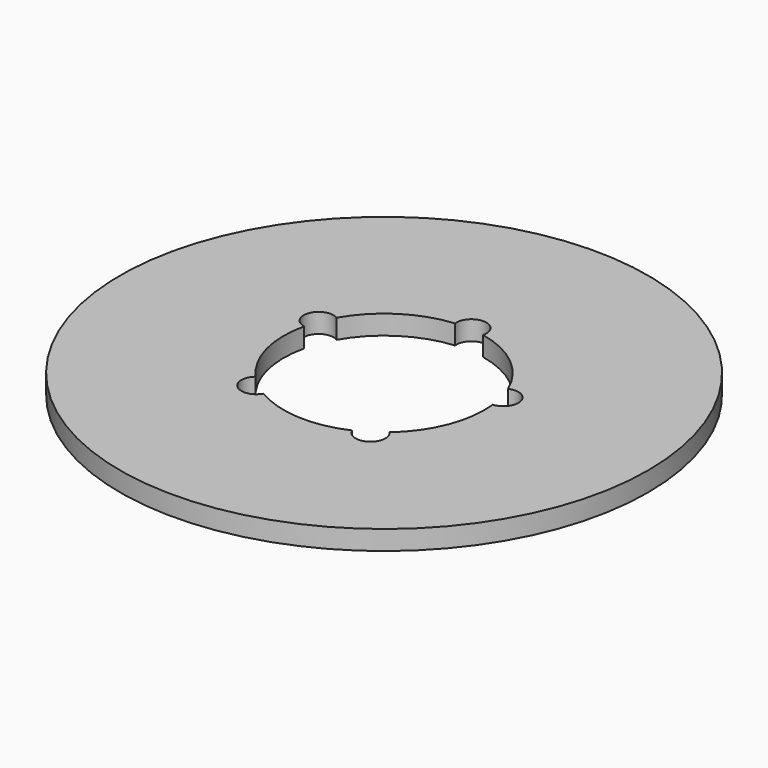
from build123d import *

# Parameters (mm, degrees)
F0_R     = 40.7341209129
F1_DEPTH = 3
F2_R     = 12.35
F3_DEPTH = 5
F4_R     = 15.5
F5_DEPTH = 3
F7_R     = 2.3
F8_DEPTH = 25


# Not quite as in the source:
# - a feature names something its author has since deleted; it is built from what else it names


with BuildPart() as f1:
    # F0 (on Top) → F1 (new body)
    with BuildSketch(Plane.XY):
        Circle(F0_R)
    extrude(amount=F1_DEPTH)

    # F2 (on face) → F3 (cut)
    with BuildSketch(Plane.XY.offset(3)):
        Circle(F2_R)
    extrude(amount=-F3_DEPTH, mode=Mode.SUBTRACT)

    # F4 (on face) → F5 (cut)
    with BuildSketch(Plane.XY.offset(3)):
        Circle(F4_R)
    extrude(amount=-F5_DEPTH, mode=Mode.SUBTRACT)

    # F7 (on face) → F8 (cut)
    with BuildSketch(Plane.XY.offset(3)):
        with Locations((15.2315180749, 3.9969421923)):
            Circle(F7_R)
        with Locations((8.4959734231, -13.2423266768)):
            Circle(F7_R)
        with Locations((-9.9757602438, -12.1809709817)):
            Circle(F7_R)
        with Locations((-14.6723501384, 5.7214666158)):
            Circle(F7_R)
        with Locations((0.8970320341, 15.7257020473)):
            Circle(F7_R)
    extrude(amount=-F8_DEPTH, mode=Mode.SUBTRACT)


solid = f1.part
